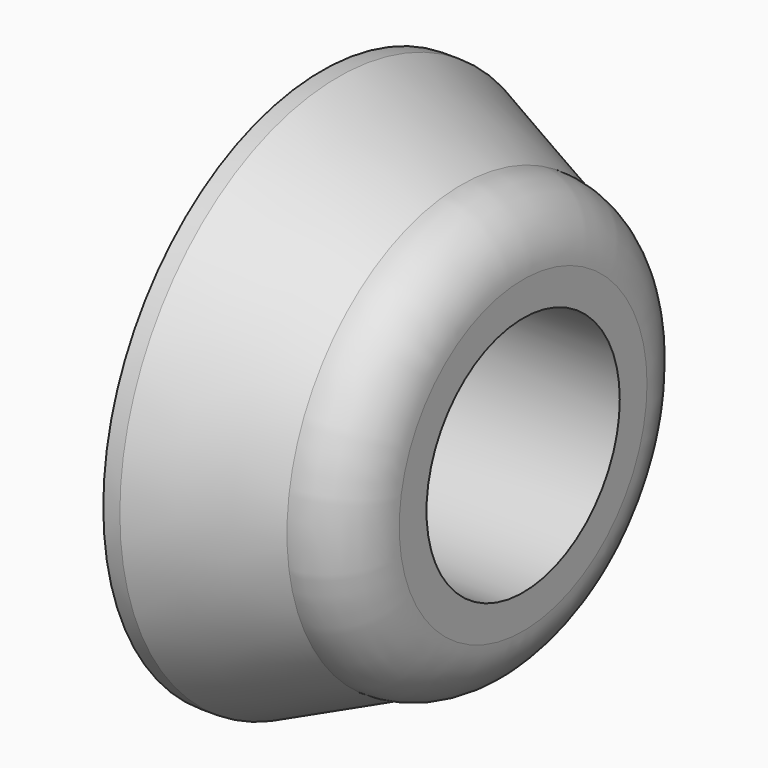
from build123d import *

# Parameters (mm, degrees)
F0_R           = 15.1824843522
F0_R_2         = 12
F1_DEPTH       = 20
F0_R_3         = 21.6830909865
F2_DEPTH       = 20
F3_R           = 6.3
F0_R_4         = 27.1312843312
F4_DEPTH       = 14
F5_S5_R        = 21.6830909865
F5_T6_DEPTH    = 40
F0_R_5         = 1.775
F6_DEPTH       = 4
F8_D           = 2.7
F8_DEPTH       = 12
F8_CSINK_D     = 7
F8_CSINK_ANGLE = 66
F8_TIP         = 0.8111618357


# Not quite as in the source:
# - a fillet or chamfer that OpenCascade refuses, or shapes differently, is made with other operations: its cross-section is extruded or revolved along the edge and cut away or added


with BuildPart() as f1:
    # F0 (on Right) → F1 (new body)
    with BuildSketch(Plane.YZ):
        Circle(F0_R)
        Circle(F0_R_2, mode=Mode.SUBTRACT)
    extrude(amount=F1_DEPTH)

    # F0 (on Right) → F2 (join)
    with BuildSketch(Plane.YZ):
        Circle(F0_R_3)
        Circle(F0_R, mode=Mode.SUBTRACT)
    extrude(amount=F2_DEPTH)

    # F3
    f3_edges = [f1.edges().sort_by_distance(p)[0] for p in [
        (20, -21.683091, 0),
    ]]
    fillet(f3_edges, radius=F3_R)

    # F0 (on Right) → F4 (join)
    with BuildSketch(Plane.YZ):
        Circle(F0_R_4)
        Circle(F0_R_3, mode=Mode.SUBTRACT)
    extrude(amount=F4_DEPTH)

    # F5: chamfer of 5.5 x 12.3532022565 on 1 edges, made by hand


with BuildPart() as f5_tool2:
    # F5_s3 → F5_t4 (revolve)
    with BuildSketch(Plane.XY):
        Polygon((14, 21.6312843312), (1.6467977435, 27.1312843312), (14, 27.1312843312), align=None)
    revolve(axis=Axis((14, 0, 0), (1, 0, 0)))

    # F5_s5 → F5_t6 (cut, symmetric)
    with BuildSketch(Plane.YZ.offset(7.8)):
        Circle(F5_S5_R)
    extrude(amount=F5_T6_DEPTH, both=True, mode=Mode.SUBTRACT)


with BuildPart() as f1_1:
    add(f1.part)

    # F5_t1: cut F5_tool2
    add(f5_tool2.part, mode=Mode.SUBTRACT)

    # F0 (on Right) → F6 (join)
    with BuildSketch(Plane.YZ):
        Circle(F0_R_2)
        Circle(F0_R_5, mode=Mode.SUBTRACT)
        Circle(F0_R_5)
    extrude(amount=F6_DEPTH)

    # F8
    with Locations(Plane.YZ.offset(4)):
        with Locations((0, 0)):
            CounterSinkHole(F8_D / 2, F8_CSINK_D / 2, depth=F8_DEPTH, counter_sink_angle=F8_CSINK_ANGLE)
            with Locations((0, 0, -(F8_DEPTH + F8_TIP / 2))):  # 118° drill point
                Cone(0, F8_D / 2, F8_TIP, mode=Mode.SUBTRACT)


solid = f1_1.part
